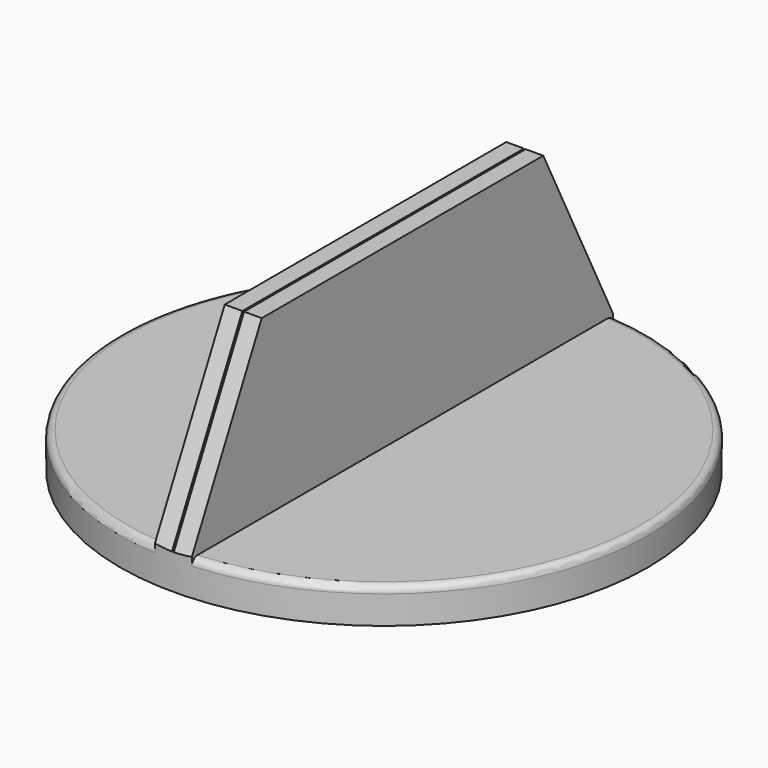
from build123d import *

# Parameters (mm, degrees)
F0_R     = 15
F1_DEPTH = 2
F3_DEPTH = 1.05
F4_DEPTH = 0.05
F5_F1_R  = 0.4
F5_F2_R  = 0.4
F0_R_2   = 19.9891271991
F6_DEPTH = 50


with BuildPart() as f1:
    # F0 (on Top) → F1 (new body)
    with BuildSketch(Plane.XY):
        Circle(F0_R)
    extrude(amount=F1_DEPTH)

    # F2 (on Right) → F3 (join, symmetric)
    with BuildSketch(Plane.YZ):
        Polygon((-10, 12), (-15, 2), (15, 2), (10, 12), align=None)
    extrude(amount=F3_DEPTH, both=True)

    # F2 (on Right) → F4 (cut, symmetric)
    with BuildSketch(Plane.YZ):
        Polygon((-10, 12), (-15, 2), (15, 2), (10, 12), align=None)
    extrude(amount=F4_DEPTH, both=True, mode=Mode.SUBTRACT)

    # F5: fillet of radius 0.4 on 3 edges, made by hand

    # F5_f1
    f5_f1_edges = [f1.edges().sort_by_distance(p)[0] for p in [
        (-15, 0, 2),
    ]]
    fillet(f5_f1_edges, radius=F5_F1_R)

    # F5_f2
    f5_f2_edges = [f1.edges().sort_by_distance(p)[0] for p in [
        (10.9715541287, 10.2286362727, 2),
        (10.9715541287, -10.2286362727, 2),
    ]]
    fillet(f5_f2_edges, radius=F5_F2_R)

    # F0 (on Top) → F6 (cut)
    with BuildSketch(Plane.XY):
        Circle(F0_R_2)
        Circle(F0_R, mode=Mode.SUBTRACT)
    extrude(amount=F6_DEPTH, mode=Mode.SUBTRACT)


solid = f1.part
